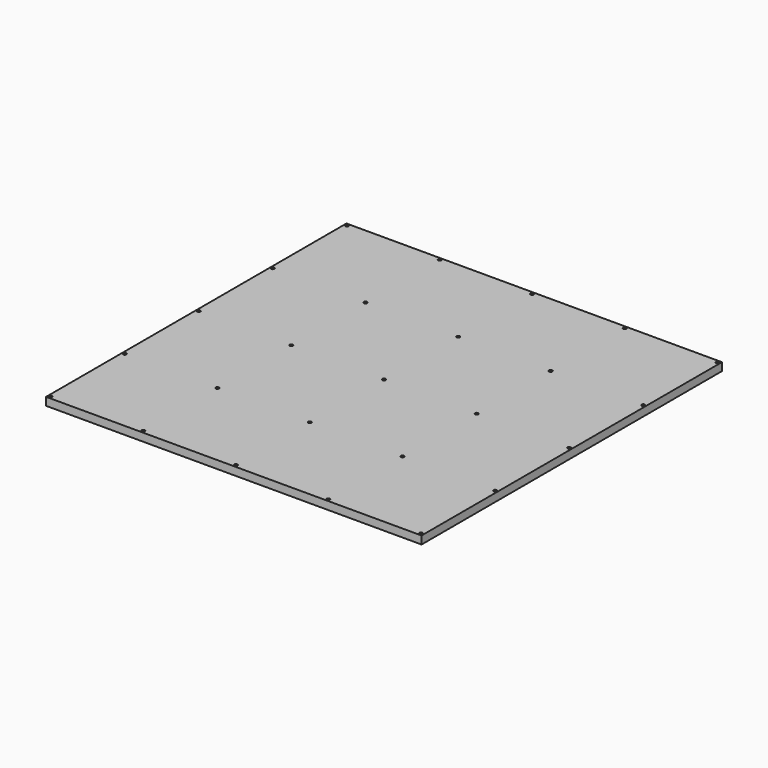
from build123d import *

# Parameters (mm, degrees)
F0_W     = 300
F0_H     = 300
F0_R     = 1.3
F1_DEPTH = 6.35


# Not quite as in the source:
# - a length typed as a fraction of an inch, garbled in the dataset ("3 / 203.2 mm" for 3/8 in), is restored


with BuildPart() as f1:
    # F0 (on Top) → F1 (new body)
    with BuildSketch(Plane.XY):
        Rectangle(F0_W, F0_H)
        with Locations((-148, -148)):
            Circle(F0_R, mode=Mode.SUBTRACT)
        with Locations((-74, -148)):
            Circle(F0_R, mode=Mode.SUBTRACT)
        with Locations((-148, -74)):
            Circle(F0_R, mode=Mode.SUBTRACT)
        with Locations((-74, -74)):
            Circle(F0_R, mode=Mode.SUBTRACT)
        with Locations((0, -148)):
            Circle(F0_R, mode=Mode.SUBTRACT)
        with Locations((74, -148)):
            Circle(F0_R, mode=Mode.SUBTRACT)
        with Locations((148, -148)):
            Circle(F0_R, mode=Mode.SUBTRACT)
        with Locations((0, -74)):
            Circle(F0_R, mode=Mode.SUBTRACT)
        with Locations((74, -74)):
            Circle(F0_R, mode=Mode.SUBTRACT)
        with Locations((148, -74)):
            Circle(F0_R, mode=Mode.SUBTRACT)
        with Locations((-148, 0)):
            Circle(F0_R, mode=Mode.SUBTRACT)
        with Locations((-148, 74)):
            Circle(F0_R, mode=Mode.SUBTRACT)
        with Locations((-74, 0)):
            Circle(F0_R, mode=Mode.SUBTRACT)
        with Locations((-74, 74)):
            Circle(F0_R, mode=Mode.SUBTRACT)
        with Locations((-148, 148)):
            Circle(F0_R, mode=Mode.SUBTRACT)
        with Locations((-74, 148)):
            Circle(F0_R, mode=Mode.SUBTRACT)
        Circle(F0_R, mode=Mode.SUBTRACT)
        with Locations((74, 0)):
            Circle(F0_R, mode=Mode.SUBTRACT)
        with Locations((0, 74)):
            Circle(F0_R, mode=Mode.SUBTRACT)
        with Locations((74, 74)):
            Circle(F0_R, mode=Mode.SUBTRACT)
        with Locations((148, 0)):
            Circle(F0_R, mode=Mode.SUBTRACT)
        with Locations((148, 74)):
            Circle(F0_R, mode=Mode.SUBTRACT)
        with Locations((0, 148)):
            Circle(F0_R, mode=Mode.SUBTRACT)
        with Locations((74, 148)):
            Circle(F0_R, mode=Mode.SUBTRACT)
        with Locations((148, 148)):
            Circle(F0_R, mode=Mode.SUBTRACT)
    extrude(amount=F1_DEPTH)


solid = f1.part
